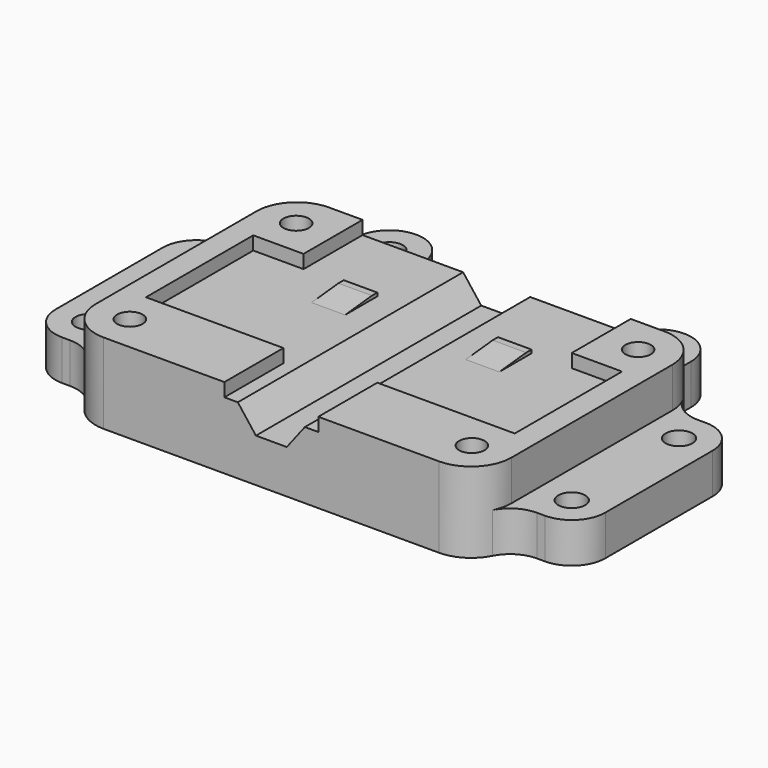
from build123d import *

# Parameters (mm, degrees)
F1_DEPTH    = 42
F4_DEPTH    = 2
F5_R        = 1.9
F6_DEPTH    = 12
F7_R        = 6
F8_W        = 30
F8_H        = 6
F9_DEPTH    = 10
F10_W       = 30
F10_H       = 6
F11_DEPTH   = 10
F12_W       = 50
F12_H       = 6
F13_DEPTH   = 10
F14_R       = 5
F15_R       = 2
F16_DEPTH   = 6
F17_W       = 5
F17_H       = 6
F18_DEPTH   = 0.5
F19_SIZE2   = 0.49999
F19_SIZE    = 4.99999
F19_2_SIZE2 = 0.49999
F19_2_SIZE  = 4.99999
F20_W       = 30
F20_H       = 10
F21_DEPTH   = 6
F22_R       = 4.99999


# Not quite as in the source:
# - a fillet or chamfer is up to 0.001 mm smaller than in the source, because OpenCascade refuses the exact size


with BuildPart() as f1:
    # F0 (on Front) → F1 (new body)
    with BuildSketch(Plane.XZ):
        Polygon((0, 10), (0, 0), (62, 0), (62, 10), (36, 10), (33.3, 6.5), (28.7, 6.5), (26, 10), align=None)
    extrude(amount=F1_DEPTH)

    # F3 (on face) → F4 (join)
    with BuildSketch(Plane.XY.offset(10)):
        Polygon((0, -42), (24, -42), (24, -31), (3.5, -31), (3.5, -11), (11, -11), (11, 0), (0, 0), align=None)
        Polygon((38, -42), (62, -42), (62, 0), (51, 0), (51, -11), (58.5, -11), (58.5, -31), (38, -31), align=None)
    extrude(amount=F4_DEPTH)

    # F5 (on face) → F6 (cut, through all)
    with BuildSketch(Plane.XY.offset(12)):
        with Locations((5.5, -5.5)):
            Circle(F5_R)
        with Locations((56.5, -5.5)):
            Circle(F5_R)
        with Locations((5.5, -36.5)):
            Circle(F5_R)
        with Locations((56.5, -36.5)):
            Circle(F5_R)
    extrude(amount=-F6_DEPTH, mode=Mode.SUBTRACT)

    # F7
    f7_edges = [f1.edges().sort_by_distance(p)[0] for p in [
        (0, -42, 6),
        (0, 0, 6),
        (62, -42, 6),
        (62, 0, 6),
    ]]
    fillet(f7_edges, radius=F7_R)

    # F8 (on face) → F9 (join)
    with BuildSketch(Plane.YZ.offset(62)):
        with Locations((-21, 3)):
            Rectangle(F8_W, F8_H)
    extrude(amount=F9_DEPTH)

    # F10 (on face) → F11 (join)
    with BuildSketch(Plane(origin=(0, 0, 0), x_dir=(0, -1, 0), z_dir=(-1, 0, 0))):
        with Locations((21, 3)):
            Rectangle(F10_W, F10_H)
    extrude(amount=F11_DEPTH)

    # F12 (on face) → F13 (join)
    with BuildSketch(Plane(origin=(0, 0, 0), x_dir=(-1, 0, 0), z_dir=(0, 1, 0))):
        with Locations((-31, 3)):
            Rectangle(F12_W, F12_H)
    extrude(amount=F13_DEPTH)

    # F14
    f14_edges = [f1.edges().sort_by_distance(p)[0] for p in [
        (6, 10, 3),
        (-10, -6, 3),
        (-10, -36, 3),
        (56, 10, 3),
        (72, -6, 3),
        (72, -36, 3),
        (6, 0, 9),
        (6, 0, 3),
        (0, -6, 9),
        (0, -6, 3),
        (0, -36, 9),
        (0, -36, 3),
        (56, 0, 9),
        (56, 0, 3),
        (62, -6, 9),
        (62, -6, 3),
        (62, -36, 3),
        (62, -36, 9),
    ]]
    fillet(f14_edges, radius=F14_R)

    # F15 (on face) → F16 (cut, through all)
    with BuildSketch(Plane.XY.offset(6)):
        with Locations((-5, -11)):
            Circle(F15_R)
        with Locations((-5, -31)):
            Circle(F15_R)
        with Locations((11, 5)):
            Circle(F15_R)
        with Locations((51, 5)):
            Circle(F15_R)
        with Locations((67, -11)):
            Circle(F15_R)
        with Locations((67, -31)):
            Circle(F15_R)
    extrude(amount=-F16_DEPTH, mode=Mode.SUBTRACT)

    # F17 (on face) → F18 (join)
    with BuildSketch(Plane.XY.offset(10)):
        with Locations((19.5, -14)):
            Rectangle(F17_W, F17_H)
        with Locations((42.5, -14)):
            Rectangle(F17_W, F17_H)
    extrude(amount=F18_DEPTH)

    # F19 (size 5 and 0.5 in the source; OpenCascade refuses exactly that, so slightly less here)
    f19_edges = [f1.edges().sort_by_distance(p)[0] for p in [
        (19.5, -17, 10.5),
    ]]
    f19_side = f1.faces().sort_by_distance((19.5, -14, 10.5))[0]
    chamfer(f19_edges, length=F19_SIZE, length2=F19_SIZE2, reference=f19_side)

    # F19#2 (size 5 and 0.5 in the source; OpenCascade refuses exactly that, so slightly less here)
    f19_2_edges = [f1.edges().sort_by_distance(p)[0] for p in [
        (42.5, -17, 10.5),
    ]]
    f19_2_side = f1.faces().sort_by_distance((42.5, -14, 10.5))[0]
    chamfer(f19_2_edges, length=F19_2_SIZE, length2=F19_2_SIZE2, reference=f19_2_side)

    # F20 (on face) → F21 (cut, through all)
    with BuildSketch(Plane.XY.offset(6)):
        with Locations((31, 5)):
            Rectangle(F20_W, F20_H)
    extrude(amount=-F21_DEPTH, mode=Mode.SUBTRACT)

    # F22 (radius 5 in the source; OpenCascade refuses exactly that, so slightly less here)
    f22_edges = [f1.edges().sort_by_distance(p)[0] for p in [
        (16, 10, 3),
        (46, 10, 3),
        (16, 0, 3),
        (46, 0, 3),
    ]]
    fillet(f22_edges, radius=F22_R)


solid = f1.part
